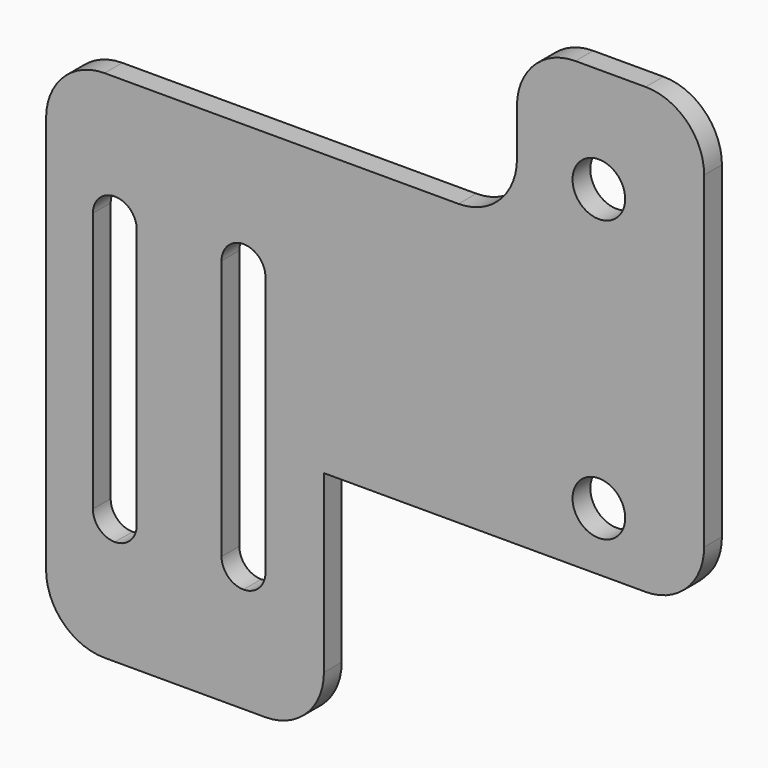
from build123d import *

# Parameters (mm, degrees)
F0_R        = 2.25
F1_DEPTH    = 1.9
F2_T1_DEPTH = 34.4776428685


# Not quite as in the source:
# - a fillet or chamfer that OpenCascade refuses, or shapes differently, is made with other operations: its cross-section is extruded or revolved along the edge and cut away or added


with BuildPart() as f1:
    # F0 (on Front) → F1 (new body)
    with BuildSketch(Plane.XZ):
        with BuildLine():
            Line((0, -33), (0, -5))
            ThreePointArc((0, -5), (-1.4644660941, -1.4644660941), (-5, 0))
            Line((-5, 0), (-11, 0))
            ThreePointArc((-11, 0), (-14.5355339059, -1.4644660941), (-16, -5))
            Line((-16, -5), (-16, -9))
            ThreePointArc((-16, -9), (-17.4644660941, -12.5355339059), (-21, -14))
            Line((-21, -14), (-51.25, -14))
            ThreePointArc((-51.25, -14), (-54.7855339059, -15.4644660941), (-56.25, -19))
            Line((-56.25, -19), (-56.25, -53))
            ThreePointArc((-56.25, -53), (-54.7855339059, -56.5355339059), (-51.25, -58))
            Line((-51.25, -58), (-37.5, -58))
            ThreePointArc((-37.5, -58), (-33.9644660941, -56.5355339059), (-32.5, -53))
            Line((-32.5, -53), (-32.5, -43))
            Line((-32.5, -43), (-32.5, -38))
            Line((-32.5, -38), (-27.5, -38))
            Line((-27.5, -38), (-5, -38))
            ThreePointArc((-5, -38), (-1.4644660941, -36.5355339059), (0, -33))
        make_face()
        with BuildLine():
            Line((-52.25, -47.125), (-52.25, -24.875))
            ThreePointArc((-52.25, -24.875), (-51.7008252147, -23.5491747853), (-50.375, -23))
            ThreePointArc((-50.375, -23), (-49.0491747853, -23.5491747853), (-48.5, -24.875))
            Line((-48.5, -24.875), (-48.5, -47.125))
            ThreePointArc((-48.5, -47.125), (-49.0491747853, -48.4508252147), (-50.375, -49))
            ThreePointArc((-50.375, -49), (-51.7008252147, -48.4508252147), (-52.25, -47.125))
        make_face(mode=Mode.SUBTRACT)
        with BuildLine():
            Line((-41.25, -47.125), (-41.25, -24.875))
            ThreePointArc((-41.25, -24.875), (-40.7008252147, -23.5491747853), (-39.375, -23))
            ThreePointArc((-39.375, -23), (-38.0491747853, -23.5491747853), (-37.5, -24.875))
            Line((-37.5, -24.875), (-37.5, -47.125))
            ThreePointArc((-37.5, -47.125), (-38.0491747853, -48.4508252147), (-39.375, -49))
            ThreePointArc((-39.375, -49), (-40.7008252147, -48.4508252147), (-41.25, -47.125))
        make_face(mode=Mode.SUBTRACT)
        with Locations((-9, -33)):
            Circle(F0_R, mode=Mode.SUBTRACT)
        with Locations((-9, -9)):
            Circle(F0_R, mode=Mode.SUBTRACT)
    extrude(amount=F1_DEPTH)

    # F2: fillet of radius 3 on 1 edges, made by hand

    # F2_s2 → F2_t1 (cut)
    with BuildSketch(Plane.YZ.offset(-32.5)):
        with BuildLine():
            ThreePointArc((-1.9, -38), (-0.5200806465, -36.8971371542), (0, -35.2089428526))
            Line((0, -35.2089428526), (0, -38))
            Line((0, -38), (-1.9, -38))
        make_face()
    extrude(amount=F2_T1_DEPTH, mode=Mode.SUBTRACT)


solid = f1.part
